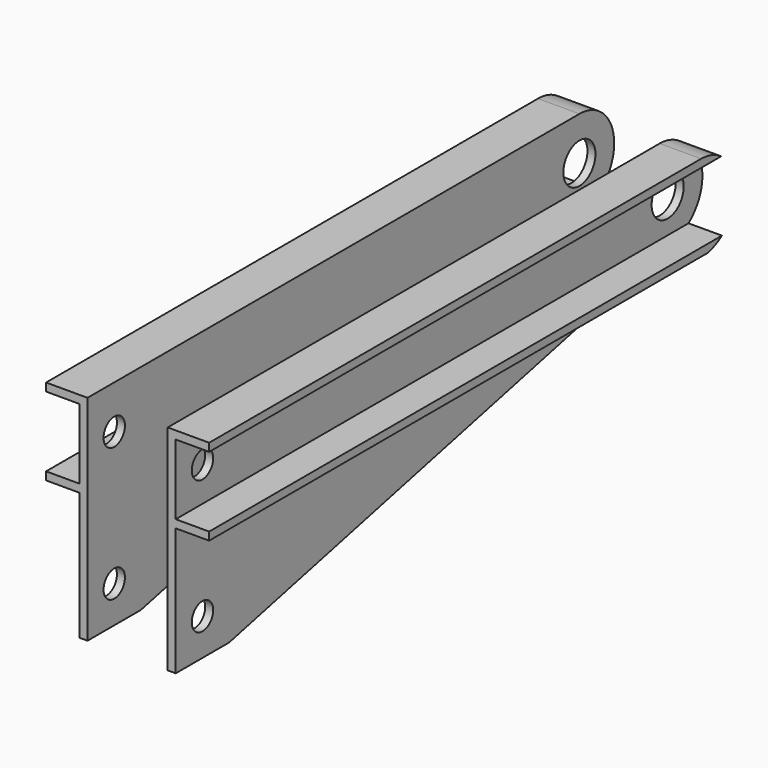
from build123d import *

# Parameters (mm, degrees)
F1_DEPTH = 100
F3_R     = 2
F3_R_2   = 3
F4_DEPTH = 12.5


# Not quite as in the source:
# - a feature names something its author has since deleted; it is built from what else it names


with BuildPart() as f1:
    # F0 (on Front) → F1 (new body)
    with BuildSketch(Plane.XZ):
        Polygon((0, 16), (0, 0), (0, -16), (1.2, -16), (1.2, 3.1), (6.2, 3.1), (6.2, 4.3), (1.2, 4.3), (1.2, 14.8), (6.2, 14.8), (6.2, 16), (1.2, 16), align=None)
    extrude(amount=-F1_DEPTH)

    # F3 (on face) → F4 (cut, symmetric)
    with BuildSketch(Plane.YZ.offset(1.2)):
        with Locations((5, -10.5)):
            Circle(F3_R)
        with Locations((5, 9.5)):
            Circle(F3_R)
        with Locations((92, 9.5)):
            Circle(F3_R_2)
        with BuildLine():
            ThreePointArc((92, 16), (98.4586436836, 10.2320667784), (93.4548179922, 3.1648990056))
            Line((93.4548179922, 3.1648990056), (10, -16))
            Line((10, -16), (100, -16))
            Line((100, -16), (100, 16))
            Line((100, 16), (92, 16))
        make_face()
    extrude(amount=F4_DEPTH, both=True, mode=Mode.SUBTRACT)


with BuildPart() as f1_1:
    # F5: moved
    add(f1.part.moved(Location((6, 0, 0))))


with BuildPart() as f6_1:
    # F6: instance of F1
    add(f1_1.part.mirror(Plane.YZ))


solid = Compound([f1_1.part, f6_1.part])
